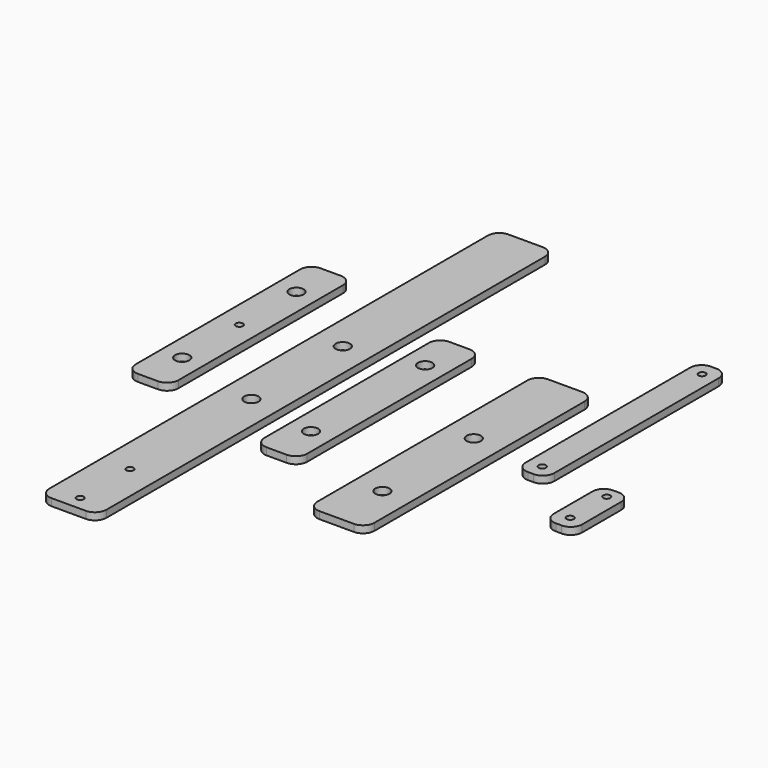
from build123d import *

# Parameters (mm, degrees)
F0_R      = 1.5875
F0_R_2    = 3.175
F6_DEPTH  = 3.175
F2_R      = 3.175
F7_DEPTH  = 3.175
F1_R      = 3.175
F8_DEPTH  = 3.175
F3_R      = 1.5875
F9_DEPTH  = 3.175
F4_R      = 3.175
F4_R_2    = 1.5875
F10_DEPTH = 3.175
F5_R      = 1.5875
F11_DEPTH = 3.175


# Not quite as in the source:
# - a length typed as a fraction of an inch, garbled in the dataset ("3 / 203.2 mm" for 3/8 in), is restored
# - a feature names something its author has since deleted; it is built from what else it names


with BuildPart() as f6:
    # F0 (on Top) → F6 (new body)
    with BuildSketch(Plane.XY):
        with BuildLine():
            Line((-125.3043544817, 177.201503253), (-140.5443544817, 177.201503253))
            ThreePointArc((-140.5443544817, 177.201503253), (-144.1364569301, 175.7136057014), (-145.6243544817, 172.121503253))
            Line((-145.6243544817, 172.121503253), (-145.6243544817, -71.718496747))
            ThreePointArc((-145.6243544817, -71.718496747), (-144.1364569301, -75.3105991954), (-140.5443544817, -76.798496747))
            Line((-140.5443544817, -76.798496747), (-125.3043544817, -76.798496747))
            ThreePointArc((-125.3043544817, -76.798496747), (-121.7122520333, -75.3105991954), (-120.2243544817, -71.718496747))
            Line((-120.2243544817, -71.718496747), (-120.2243544817, 172.121503253))
            ThreePointArc((-120.2243544817, 172.121503253), (-121.7122520333, 175.7136057014), (-125.3043544817, 177.201503253))
        make_face()
        with Locations((-132.9243544817, -70.448496747)):
            Circle(F0_R, mode=Mode.SUBTRACT)
        with Locations((-132.948756218, -42.686296747)):
            Circle(F0_R, mode=Mode.SUBTRACT)
        with Locations((-132.9243544817, 24.801503253)):
            Circle(F0_R_2, mode=Mode.SUBTRACT)
        with Locations((-132.9243544817, 75.601503253)):
            Circle(F0_R_2, mode=Mode.SUBTRACT)
    extrude(amount=F6_DEPTH)


with BuildPart() as f7:
    # F2 (on Top) → F7 (new body)
    with BuildSketch(Plane.XY):
        with BuildLine():
            Line((-97.1865381289, 101.3134590626), (-106.0765381289, 101.3134590626))
            ThreePointArc((-106.0765381289, 101.3134590626), (-109.6686405773, 99.825561511), (-111.1565381289, 96.2334590626))
            Line((-111.1565381289, 96.2334590626), (-111.1565381289, 4.7934590626))
            ThreePointArc((-111.1565381289, 4.7934590626), (-109.6686405773, 1.2013566141), (-106.0765381289, -0.2865409374))
            Line((-106.0765381289, -0.2865409374), (-97.1865381289, -0.2865409374))
            ThreePointArc((-97.1865381289, -0.2865409374), (-93.5944356804, 1.2013566141), (-92.1065381289, 4.7934590626))
            Line((-92.1065381289, 4.7934590626), (-92.1065381289, 96.2334590626))
            ThreePointArc((-92.1065381289, 96.2334590626), (-93.5944356804, 99.825561511), (-97.1865381289, 101.3134590626))
        make_face()
        with Locations((-101.6315381289, 18.7634590626)):
            Circle(F2_R, mode=Mode.SUBTRACT)
        with Locations((-101.6315381289, 82.2634590626)):
            Circle(F2_R, mode=Mode.SUBTRACT)
    extrude(amount=F7_DEPTH)


with BuildPart() as f8:
    # F1 (on Top) → F8 (new body)
    with BuildSketch(Plane.XY):
        with BuildLine():
            Line((-46.4988631535, 100.7131136298), (-61.7388631535, 100.7131136298))
            ThreePointArc((-61.7388631535, 100.7131136298), (-65.3309656019, 99.2252160782), (-66.8188631535, 95.6331136298))
            Line((-66.8188631535, 95.6331136298), (-66.8188631535, -21.2068863702))
            ThreePointArc((-66.8188631535, -21.2068863702), (-65.3309656019, -24.7989888186), (-61.7388631535, -26.2868863702))
            Line((-61.7388631535, -26.2868863702), (-46.4988631535, -26.2868863702))
            ThreePointArc((-46.4988631535, -26.2868863702), (-42.906760705, -24.7989888186), (-41.4188631535, -21.2068863702))
            Line((-41.4188631535, -21.2068863702), (-41.4188631535, 95.6331136298))
            ThreePointArc((-41.4188631535, 95.6331136298), (-42.906760705, 99.2252160782), (-46.4988631535, 100.7131136298))
        make_face()
        with Locations((-54.1188631535, -0.8868863702)):
            Circle(F1_R, mode=Mode.SUBTRACT)
        with Locations((-54.1188631535, 49.9131136298)):
            Circle(F1_R, mode=Mode.SUBTRACT)
    extrude(amount=F8_DEPTH)


with BuildPart() as f9:
    # F3 (on Top) → F9 (new body)
    with BuildSketch(Plane.XY):
        with BuildLine():
            Line((-21.075289588, 143.5134345447), (-23.615289588, 143.5134345447))
            ThreePointArc((-23.615289588, 143.5134345447), (-27.2073920364, 142.0255369931), (-28.695289588, 138.4334345447))
            Line((-28.695289588, 138.4334345447), (-28.695289588, 46.9934345447))
            ThreePointArc((-28.695289588, 46.9934345447), (-27.2073920364, 43.4013320963), (-23.615289588, 41.9134345447))
            Line((-23.615289588, 41.9134345447), (-21.075289588, 41.9134345447))
            ThreePointArc((-21.075289588, 41.9134345447), (-17.4831871395, 43.4013320963), (-15.995289588, 46.9934345447))
            Line((-15.995289588, 46.9934345447), (-15.995289588, 138.4334345447))
            ThreePointArc((-15.995289588, 138.4334345447), (-17.4831871395, 142.0255369931), (-21.075289588, 143.5134345447))
        make_face()
        with Locations((-22.345289588, 48.2634345447)):
            Circle(F3_R, mode=Mode.SUBTRACT)
        with Locations((-22.3452951759, 137.1634345447)):
            Circle(F3_R, mode=Mode.SUBTRACT)
    extrude(amount=F9_DEPTH)


with BuildPart() as f10:
    # F4 (on Top) → F10 (new body)
    with BuildSketch(Plane.XY):
        with BuildLine():
            Line((-166.6488225746, 116.5749058127), (-175.5388225746, 116.5749058127))
            ThreePointArc((-175.5388225746, 116.5749058127), (-179.130925023, 115.0870082612), (-180.6188225746, 111.4949058127))
            Line((-180.6188225746, 111.4949058127), (-180.6188225746, 20.0549058127))
            ThreePointArc((-180.6188225746, 20.0549058127), (-179.130925023, 16.4628033643), (-175.5388225746, 14.9749058127))
            Line((-175.5388225746, 14.9749058127), (-166.6488225746, 14.9749058127))
            ThreePointArc((-166.6488225746, 14.9749058127), (-163.0567201262, 16.4628033643), (-161.5688225746, 20.0549058127))
            Line((-161.5688225746, 20.0549058127), (-161.5688225746, 111.4949058127))
            ThreePointArc((-161.5688225746, 111.4949058127), (-163.0567201262, 115.0870082612), (-166.6488225746, 116.5749058127))
        make_face()
        with Locations((-171.0938225746, 34.0249058127)):
            Circle(F4_R, mode=Mode.SUBTRACT)
        with Locations((-171.0938225746, 65.7749058127)):
            Circle(F4_R_2, mode=Mode.SUBTRACT)
        with Locations((-171.0938225746, 97.5249058127)):
            Circle(F4_R, mode=Mode.SUBTRACT)
    extrude(amount=F10_DEPTH)


with BuildPart() as f11:
    # F5 (on Top) → F11 (new body)
    with BuildSketch(Plane.XY):
        with BuildLine():
            Line((10.6020793927, 49.5937959403), (8.0620793927, 49.5937959403))
            ThreePointArc((8.0620793927, 49.5937959403), (4.4699769443, 48.1058983887), (2.9820793927, 44.5137959403))
            Line((2.9820793927, 44.5137959403), (2.9820793927, 22.9237959403))
            ThreePointArc((2.9820793927, 22.9237959403), (4.4699769443, 19.3316934919), (8.0620793927, 17.8437959403))
            Line((8.0620793927, 17.8437959403), (10.6020793927, 17.8437959403))
            ThreePointArc((10.6020793927, 17.8437959403), (14.1941818412, 19.3316934919), (15.6820793927, 22.9237959403))
            Line((15.6820793927, 22.9237959403), (15.6820793927, 44.5137959403))
            ThreePointArc((15.6820793927, 44.5137959403), (14.1941818412, 48.1058983887), (10.6020793927, 49.5937959403))
        make_face()
        with Locations((9.3320793927, 24.1937959403)):
            Circle(F5_R, mode=Mode.SUBTRACT)
        with Locations((9.3320793927, 44.5137959403)):
            Circle(F5_R, mode=Mode.SUBTRACT)
    extrude(amount=F11_DEPTH)


solid = Compound([f6.part, f7.part, f8.part, f9.part, f10.part, f11.part])
